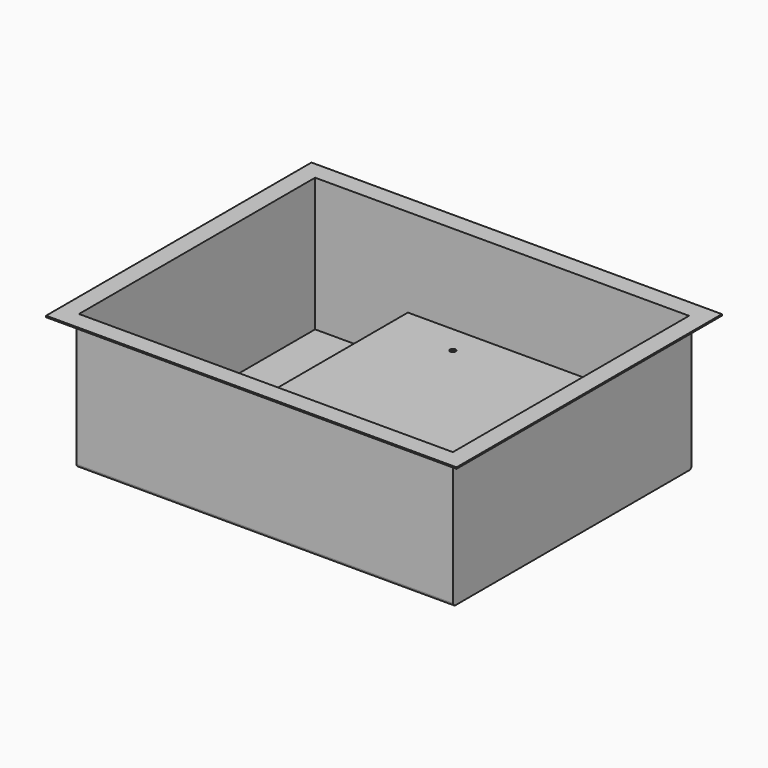
from build123d import *

# Parameters (mm, degrees)
F0_W      = 850.9
F0_H      = 673.1
F1_DEPTH  = 304.8
F2_T      = -3.175
F3_W      = 584.2
F3_H      = 101.6
F4_DEPTH  = 558.8
F5_W      = 431.8
F5_H      = 69.85
F6_DEPTH  = 25.4
F7_T      = -2.54
F8_R      = 6.35
F9_DEPTH  = 2.54
F10_W     = 927.1
F10_H     = 749.3
F10_W_2   = 850.9
F10_H_2   = 673.1
F11_DEPTH = 3.175
F12_R     = 6.35
F13_R     = 6.35
F15_DEPTH = 584.2


# Not quite as in the source:
# - a shell that OpenCascade refuses in one call is made with other operations: the cavity is built on its own and cut out


with BuildPart() as f1:
    # F0 (on Top) → F1 (new body)
    with BuildSketch(Plane.XY):
        Rectangle(F0_W, F0_H)
    extrude(amount=F1_DEPTH)

    # F2
    f2_openings = [f1.faces().sort_by_distance(p)[0] for p in [
        (0, 0, 304.8),
    ]]
    offset(amount=F2_T, openings=f2_openings)

    # F3 (on face) → F4 (join)
    with BuildSketch(Plane.XZ.offset(-333.375)):
        with Locations((79.3750111103, 53.975)):
            Rectangle(F3_W, F3_H)
    extrude(amount=F4_DEPTH)

    # F5 (on face) → F6 (cut)
    with BuildSketch(Plane.XZ.offset(225.425)):
        with Locations((79.3750111103, 38.1)):
            Rectangle(F5_W, F5_H)
    extrude(amount=-F6_DEPTH, mode=Mode.SUBTRACT)

    # F7: a shell. OpenCascade refuses it in one call, so the cavity is built on its own and cut out:
    # the body offset inwards by the wall thickness, plus a prism from it out through each open face.
    f7_core = offset(f1.part, amount=F7_T, kind=Kind.INTERSECTION, mode=Mode.PRIVATE)
    f7_exits = [f7_core.faces().sort_by_distance(p)[0] for p in [
        (303.691397, -222.885, 39.0525),
    ]]
    add(f7_core, mode=Mode.SUBTRACT)
    extrude(f7_exits, amount=-F7_T, mode=Mode.SUBTRACT)

    # F8 (on face) → F9 (cut, through all)
    with BuildSketch(Plane.XY.offset(104.775)):
        with Locations((219.0750111103, 269.875)):
            Circle(F8_R)
        with Locations((-60.3249888897, 269.875)):
            Circle(F8_R)
        with Locations((-60.3249888897, -161.925)):
            Circle(F8_R)
        with Locations((219.0750111103, -161.925)):
            Circle(F8_R)
    extrude(amount=-F9_DEPTH, mode=Mode.SUBTRACT)

    # F10 (on face) → F11 (join)
    with BuildSketch(Plane.XY.offset(304.8)):
        Rectangle(F10_W, F10_H)
        Rectangle(F10_W_2, F10_H_2, mode=Mode.SUBTRACT)
    extrude(amount=-F11_DEPTH)

    # F12
    f12_edges = [f1.edges().sort_by_distance(p)[0] for p in [
        (0, -336.55, 0),
    ]]
    fillet(f12_edges, radius=F12_R)

    # F13
    f13_edges = [f1.edges().sort_by_distance(p)[0] for p in [
        (0, 336.55, 0),
    ]]
    fillet(f13_edges, radius=F13_R)

    # F14 (on face) → F15 (cut, through all)
    with BuildSketch(Plane(origin=(-212.7249888897, 0, 0), x_dir=(0, -1, 0), z_dir=(-1, 0, 0))):
        with BuildLine():
            ThreePointArc((-254.2258527756, 3.175), (-277.4081012725, 59.1418987275), (-333.375, 82.3241472244))
            Line((-333.375, 82.3241472244), (-333.375, 3.175))
            Line((-333.375, 3.175), (-254.2258527756, 3.175))
        make_face()
    extrude(amount=-F15_DEPTH, mode=Mode.SUBTRACT)


solid = f1.part
